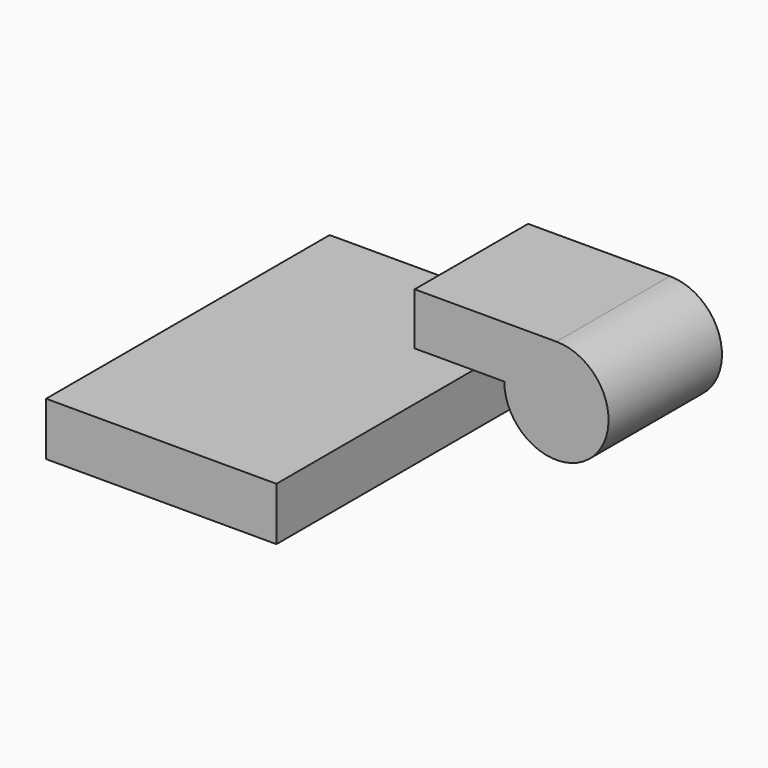
from build123d import *

# Parameters (mm, degrees)
F1_DEPTH  = 63.5
F0_W      = 50.8
F0_H      = 18.669
F2_DEPTH  = 25.4
F2_FACE_W = 50.8
F2_FACE_H = 18.669


with BuildPart() as f1:
    # F0 (on Front) → F1 (new body, symmetric)
    with BuildSketch(Plane.XZ):
        Polygon((22.225, 3.9350592289), (-41.275, 3.9350592289), (-41.275, -15.1149407711), (41.275, -15.1149407711), (41.275, 3.9350592289), align=None)
    extrude(amount=F1_DEPTH, both=True)


with BuildPart() as f2:
    # F0 (on Front) → F2 (new body, symmetric)
    with BuildSketch(Plane.XZ):
        with Locations((85.725, 46.6705592289)):
            Rectangle(F0_W, F0_H)
    extrude(amount=F2_DEPTH, both=True)

    # F2_face (on face) → F3 (revolve)
    with BuildSketch(Plane(origin=(111.125, 0, 46.6705592289), x_dir=(0, 1, 0), z_dir=(1, 0, 0))):
        Rectangle(F2_FACE_W, F2_FACE_H)
    revolve(axis=Axis((111.125, 0, 37.3360592289), (0, 1, 0)))


solid = Compound([f1.part, f2.part])
